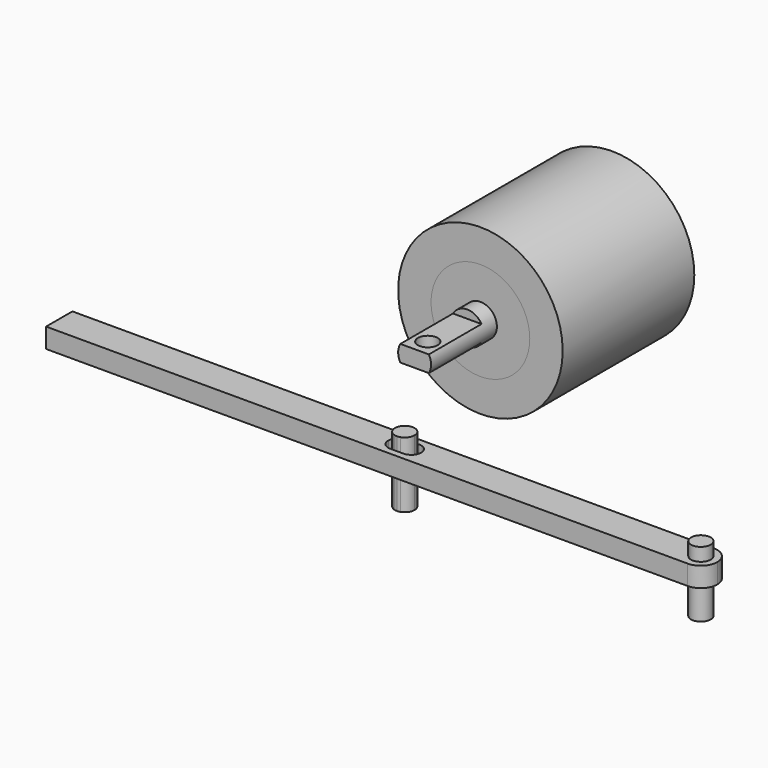
from build123d import *

# Parameters (mm, degrees)
F0_R      = 1.5
F1_DEPTH  = 3
F2_DEPTH  = 5
F4_R      = 12.5
F4_R_2    = 7.5
F5_DEPTH  = 12.5
F4_R_3    = 2.5
F6_DEPTH  = 12.5
F7_DEPTH  = 25
F9_DEPTH  = 10
F10_R     = 1.5
F11_DEPTH = 25


# Not quite as in the source:
# - a feature names something its author has since deleted; it is built from what else it names


with BuildPart() as f1:
    # F0 (on Top) → F1 (new body)
    with BuildSketch(Plane.XY):
        with BuildLine():
            ThreePointArc((47.5, -2.5), (45, 0), (47.5, 2.5))
            Line((47.5, 2.5), (-50, 2.5))
            Line((-50, 2.5), (-50, -2.5))
            Line((-50, -2.5), (47.5, -2.5))
        make_face()
        Polygon((1.5, 1.5), (2.5, 1.5), (3.5, 1.5), (5, 1.5), (5, 0), (5, -1.5), (3.5, -1.5), (2.5, -1.5), (1.5, -1.5), (0, -1.5), (0, 0), (0, 1.5), align=None, mode=Mode.SUBTRACT)
        with BuildLine():
            ThreePointArc((50, 0), (49.267766953, 1.767766953), (47.5, 2.5))
            ThreePointArc((47.5, 2.5), (45, 0), (47.5, -2.5))
            ThreePointArc((47.5, -2.5), (49.267766953, -1.767766953), (50, 0))
        make_face()
        with Locations((47.5, 0)):
            Circle(F0_R, mode=Mode.SUBTRACT)
        with BuildLine():
            ThreePointArc((0, 0), (0.4393398282, 1.0606601718), (1.5, 1.5))
            Line((1.5, 1.5), (0, 1.5))
            Line((0, 1.5), (0, 0))
        make_face()
        with BuildLine():
            Line((0, -1.5), (1.5, -1.5))
            ThreePointArc((1.5, -1.5), (0.4393398282, -1.0606601718), (0, 0))
            Line((0, 0), (0, -1.5))
        make_face()
        with BuildLine():
            ThreePointArc((5, 0), (4.5606601718, -1.0606601718), (3.5, -1.5))
            Line((3.5, -1.5), (5, -1.5))
            Line((5, -1.5), (5, 0))
        make_face()
        with BuildLine():
            Line((5, 1.5), (3.5, 1.5))
            ThreePointArc((3.5, 1.5), (4.5606601718, 1.0606601718), (5, 0))
            Line((5, 0), (5, 1.5))
        make_face()
    extrude(amount=F1_DEPTH)


with BuildPart() as f2:
    # F0 (on Top) → F2 (new body, symmetric)
    with BuildSketch(Plane.XY):
        with BuildLine():
            ThreePointArc((2.5, 1.1180339887), (2.7355194018, 1.290569415), (3, 1.4142135624))
            ThreePointArc((3, 1.4142135624), (2.7536529681, 1.4783978395), (2.5, 1.5))
            ThreePointArc((2.5, 1.5), (2.2463470319, 1.4783978395), (2, 1.4142135624))
            ThreePointArc((2, 1.4142135624), (2.2644805982, 1.290569415), (2.5, 1.1180339887))
        make_face()
        with BuildLine():
            ThreePointArc((2.5, -1.5), (2.7536529681, -1.4783978395), (3, -1.4142135624))
            ThreePointArc((3, -1.4142135624), (2.7355194018, -1.290569415), (2.5, -1.1180339887))
            ThreePointArc((2.5, -1.1180339887), (2.2644805982, -1.290569415), (2, -1.4142135624))
            ThreePointArc((2, -1.4142135624), (2.2463470319, -1.4783978395), (2.5, -1.5))
        make_face()
        with BuildLine():
            ThreePointArc((2.5, -1.1180339887), (2, 0), (2.5, 1.1180339887))
            ThreePointArc((2.5, 1.1180339887), (2.2644805982, 1.290569415), (2, 1.4142135624))
            ThreePointArc((2, 1.4142135624), (1, 0), (2, -1.4142135624))
            ThreePointArc((2, -1.4142135624), (2.2644805982, -1.290569415), (2.5, -1.1180339887))
        make_face()
        with BuildLine():
            ThreePointArc((3, -1.4142135624), (3.7247448714, -0.8660254038), (4, 0))
            ThreePointArc((4, 0), (3.7247448714, 0.8660254038), (3, 1.4142135624))
            ThreePointArc((3, 1.4142135624), (2.7355194018, 1.290569415), (2.5, 1.1180339887))
            ThreePointArc((2.5, 1.1180339887), (2.8693063938, 0.6123724357), (3, 0))
            ThreePointArc((3, 0), (2.8693063938, -0.6123724357), (2.5, -1.1180339887))
            ThreePointArc((2.5, -1.1180339887), (2.7355194018, -1.290569415), (3, -1.4142135624))
        make_face()
        with BuildLine():
            ThreePointArc((3, 0), (2.8693063938, 0.6123724357), (2.5, 1.1180339887))
            ThreePointArc((2.5, 1.1180339887), (2, 0), (2.5, -1.1180339887))
            ThreePointArc((2.5, -1.1180339887), (2.8693063938, -0.6123724357), (3, 0))
        make_face()
    extrude(amount=F2_DEPTH, both=True)


with BuildPart() as f2b:
    # F0 (on Top) → F2, piece 2 (new body, symmetric)
    with BuildSketch(Plane.XY):
        with Locations((47.5, 0)):
            Circle(F0_R)
    extrude(amount=F2_DEPTH, both=True)


with BuildPart() as f5:
    # F4 (on offset) → F5 (new body, symmetric)
    with BuildSketch(Plane.XZ.offset(-30)):
        with Locations((0, 11.9395209476)):
            Circle(F4_R)
        with Locations((0, 11.9395209476)):
            Circle(F4_R_2, mode=Mode.SUBTRACT)
    extrude(amount=F5_DEPTH, both=True)


with BuildPart() as f6:
    # F4 (on offset) → F6 (new body, symmetric)
    with BuildSketch(Plane.XZ.offset(-30)):
        with Locations((0, 11.9395209476)):
            Circle(F4_R_2)
        with Locations((0, 11.9395209476)):
            Circle(F4_R_3, mode=Mode.SUBTRACT)
    extrude(amount=F6_DEPTH, both=True)

    # F4 (on offset) → F7 (join)
    with BuildSketch(Plane.XZ.offset(-30)):
        with Locations((0, 11.9395209476)):
            Circle(F4_R_3)
    extrude(amount=F7_DEPTH)

    # F8 (on face) → F9 (cut)
    with BuildSketch(Plane.XZ.offset(-5)):
        with BuildLine():
            ThreePointArc((-2.1650635095, 10.6895209476), (0, 9.4395209476), (2.1650635095, 10.6895209476))
            Line((2.1650635095, 10.6895209476), (-2.1650635095, 10.6895209476))
        make_face()
        with BuildLine():
            Line((-2.1650635095, 13.1895209476), (2.1650635095, 13.1895209476))
            ThreePointArc((2.1650635095, 13.1895209476), (0, 14.4395209476), (-2.1650635095, 13.1895209476))
        make_face()
    extrude(amount=-F9_DEPTH, mode=Mode.SUBTRACT)

    # F10 (on face) → F11 (cut)
    with BuildSketch(Plane(origin=(0, 0, 10.6895209476), x_dir=(1, 0, 0), z_dir=(0, 0, -1))):
        with Locations((0, -7.5)):
            Circle(F10_R)
    extrude(amount=-F11_DEPTH, mode=Mode.SUBTRACT)


solid = Compound([f1.part, f2.part, f2b.part, f5.part, f6.part])
